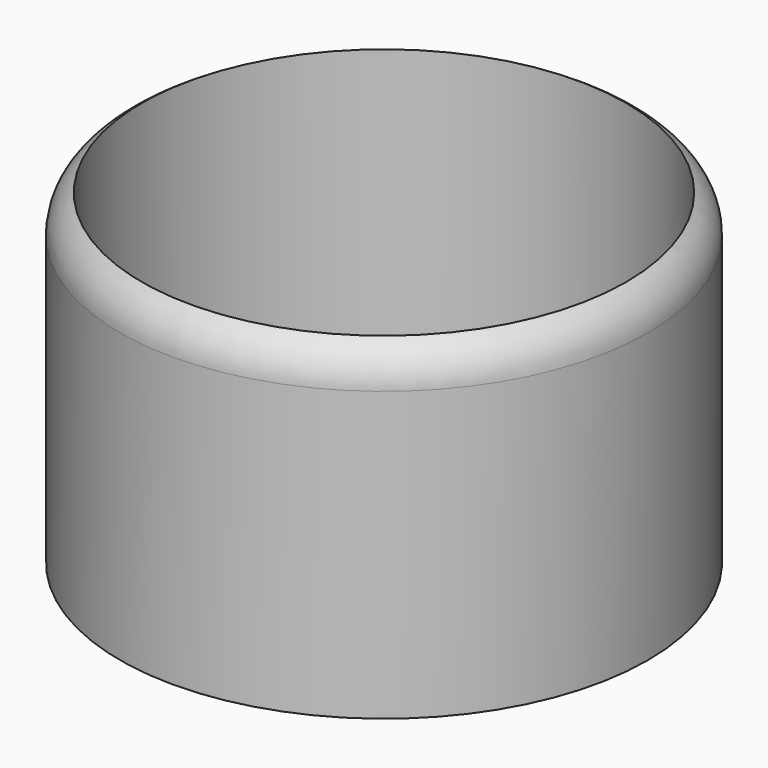
from build123d import *

# Parameters (mm, degrees)
F0_R     = 30.8666383599
F1_DEPTH = 19.05
F2_T     = -2.54


# Not quite as in the source:
# - a fillet or chamfer that OpenCascade refuses, or shapes differently, is made with other operations: its cross-section is extruded or revolved along the edge and cut away or added


with BuildPart() as f1:
    # F0 (on Top) → F1 (new body, symmetric)
    with BuildSketch(Plane.XY):
        Circle(F0_R)
    extrude(amount=F1_DEPTH, both=True)

    # F2
    f2_openings = [f1.faces().sort_by_distance(p)[0] for p in [
        (0, 0, 19.05),
    ]]
    offset(amount=F2_T, openings=f2_openings)

    # F3: fillet of radius 5.08 on 1 edges, made by hand

    # F3_s1 → F3_t2 (revolve, cut)
    with BuildSketch(Plane.XZ):
        with BuildLine():
            ThreePointArc((30.8666383599, 14.6505909488), (30.1860474111, 17.1905909488), (28.3266383599, 19.05))
            Line((28.3266383599, 19.05), (28.3774383599, 19.137988181))
            ThreePointArc((28.3774383599, 19.137988181), (29.5966383599, 19.1516), (30.8666383599, 19.1516))
            Line((30.8666383599, 19.1516), (30.9682383599, 19.05))
            Line((30.9682383599, 19.05), (30.9682383599, 14.6505909488))
            Line((30.9682383599, 14.6505909488), (30.8666383599, 14.6505909488))
        make_face()
    revolve(axis=Axis((0, 0, 19.05), (0, 0, 1)), mode=Mode.SUBTRACT)


solid = f1.part
